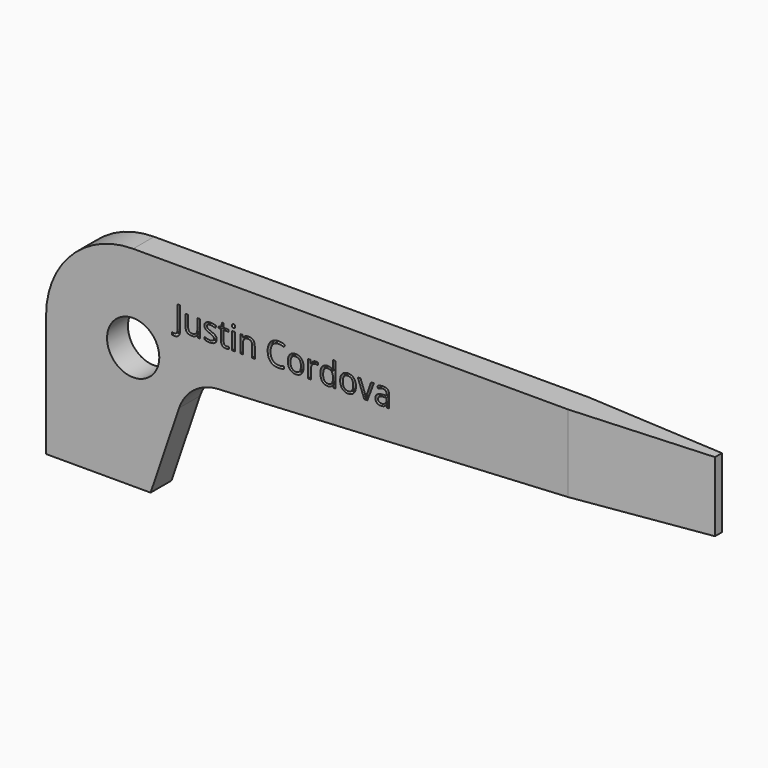
from build123d import *

# Parameters (mm, degrees)
F1_DEPTH     = 2.38125
F2_R         = 2.38125
F3_DEPTH     = 2.38225
F5_DEPTH     = 25.4
F6_TEXT_SIZE = 2.9331409476
F7_DEPTH     = 0.508


# Not quite as in the source:
# - Text() gives the source's letters only with a copy of the font that has no kerning and outlines rounded to 1/6400 em; it was checked with that copy


with BuildPart() as f1:
    # F0 (on Front) → F1 (new body)
    with BuildSketch(Plane.XZ):
        with BuildLine():
            Line((60.325, 19.05), (7.9375, 19.05))
            ThreePointArc((7.9375, 19.05), (2.3248399243, 16.7251600757), (0, 11.1125))
            Line((0, 11.1125), (0, 0))
            Line((0, 0), (9.525, 0))
            Line((9.525, 0), (12.1173647876, 7.6271664624))
            ThreePointArc((12.1173647876, 7.6271664624), (13.4786145605, 9.5135918491), (15.6631963617, 10.3130942181))
            Line((15.6631963617, 10.3130942181), (60.325, 12.7))
            Line((60.325, 12.7), (60.325, 19.05))
        make_face()
    extrude(amount=F1_DEPTH)

    # F2 (on face) → F3 (cut, through all)
    with BuildSketch(Plane.XZ.offset(2.38125)):
        with Locations((7.9375, 11.1125)):
            Circle(F2_R)
    extrude(amount=-F3_DEPTH, mode=Mode.SUBTRACT)

    # F4 (on face) → F5 (cut)
    with BuildSketch(Plane.XY.offset(19.05)):
        Polygon((60.325, -2.38125), (60.325, -1.5875), (47.5597642362, -2.38125), align=None)
        Polygon((60.325, 0), (47.5597642362, 0), (60.325, -0.79375), align=None)
    extrude(amount=-F5_DEPTH, mode=Mode.SUBTRACT)

    # F6 (on face) → F7 (cut)
    with BuildSketch(Plane.XZ.offset(2.38125)):
        with Locations((11.6945421323, 13.8265527785)):
            Text('Justin Cordova', F6_TEXT_SIZE, font='Open Sans', text_align=(TextAlign.LEFT, TextAlign.BOTTOM))
    extrude(amount=-F7_DEPTH, mode=Mode.SUBTRACT)


solid = f1.part
